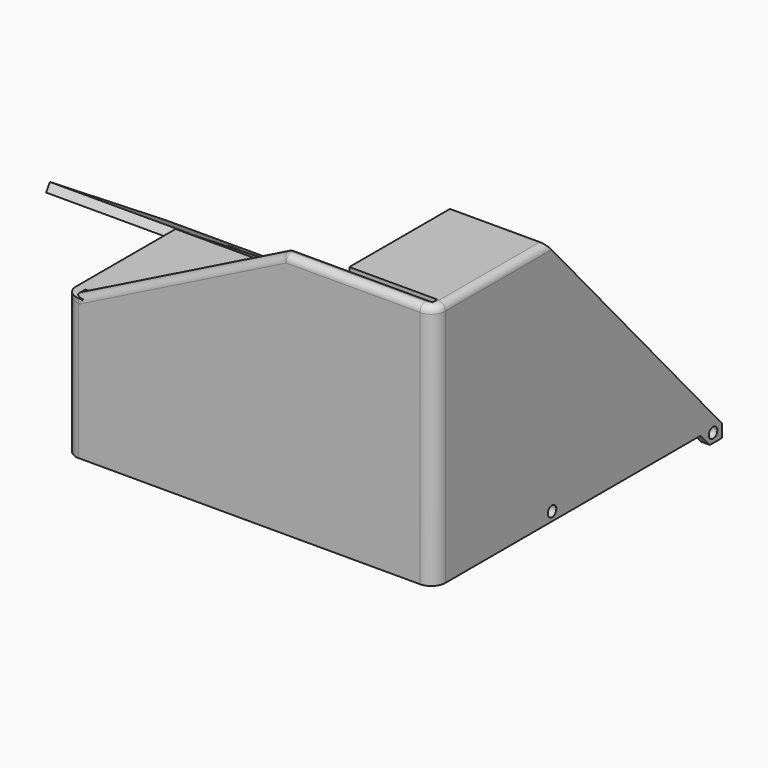
from build123d import *

# Parameters (mm, degrees)
F1_DEPTH      = 3.175
F2_R          = 1.905
F3_DEPTH      = 3.175
F4_R          = 5.08
F5_W          = 45.4158770088
F5_H          = 3.3436195493
F6_DEPTH      = 31.75
F8_DEPTH      = 3.175
F9_W          = 44.698641931
F9_H          = 3.175
F10_DEPTH     = 31.75
F11_R         = 5.08
F13_DEPTH     = 50.8
F14_R         = 1.905
F15_DEPTH     = 25.4
F16_R         = 1.905
F17_DEPTH     = 25.4
F18_T4_DEPTH  = 95.7643351942
F18_T9_DEPTH  = 95.7643351942
F18_S10_R     = 5.08
F18_T11_DEPTH = 50
F19_T1_DEPTH  = 48.2953873372
F19_T3_DEPTH  = 52.07
F19_T5_DEPTH  = 2.1340316571
F19_T10_DEPTH = 2.54
F19_T14_ANGLE = 90


# Not quite as in the source:
# - a fillet or chamfer that OpenCascade refuses, or shapes differently, is made with other operations: its cross-section is extruded or revolved along the edge and cut away or added


with BuildPart() as f1:
    # F0 (on Front) → F1 (new body)
    with BuildSketch(Plane.XZ):
        Polygon((-76.2, 0), (0, 0), (50.8, 0), (50.8, 88.9), (0, 88.9), (-76.2, 50.8), align=None)
    extrude(amount=F1_DEPTH)

    # F2 (on face) → F3 (join)
    with BuildSketch(Plane.YZ.offset(50.8)):
        Polygon((47.625, 88.9), (-3.175, 88.9), (-3.175, 0), (117.0480847359, 0), (121.2547570467, -4.6795206144), (126.6633123159, -4.6795206144), (126.6633123159, 0), align=None)
        with Locations((50.0349625945, 3.2108949963)):
            Circle(F2_R, mode=Mode.SUBTRACT)
        with Locations((122.6691529155, -1.3459949987)):
            Circle(F2_R, mode=Mode.SUBTRACT)
    extrude(amount=F3_DEPTH)

    # F4
    f4_edges = [f1.edges().sort_by_distance(p)[0] for p in [
        (53.975, -3.175, 44.45),
    ]]
    fillet(f4_edges, radius=F4_R)

    # F5 (on face) → F6 (join)
    with BuildSketch(Plane(origin=(50.8, 0, 0), x_dir=(0, -1, 0), z_dir=(-1, 0, 0))):
        with Locations((-24.9170614956, 87.2281902254)):
            Rectangle(F5_W, F5_H)
    extrude(amount=F6_DEPTH)

    # F7 (on face) → F8 (join)
    with BuildSketch(Plane(origin=(-76.2, 0, 0), x_dir=(0, -1, 0), z_dir=(-1, 0, 0))):
        Polygon((-46.908441931, 50.8), (-126.4358460903, 0), (-126.4358460903, -4.5622045459), (-121.1352100604, -4.5622045459), (-113.9930784702, 0), (3.175, 0), (3.175, 50.8), align=None)
    extrude(amount=F8_DEPTH)

    # F9 (on face) → F10 (join)
    with BuildSketch(Plane.YZ.offset(-76.2)):
        with Locations((24.5591209655, 49.2125)):
            Rectangle(F9_W, F9_H)
    extrude(amount=F10_DEPTH)

    # F11
    f11_edges = [f1.edges().sort_by_distance(p)[0] for p in [
        (-79.375, -3.175, 25.4),
    ]]
    fillet(f11_edges, radius=F11_R)

    # F12 (on face) → F13 (join)
    with BuildSketch(Plane(origin=(-79.375, 0, 0), x_dir=(0, -1, 0), z_dir=(-1, 0, 0))):
        Polygon((-51.9476211918, 43.8136345955), (-53.6567879294, 46.4893352632), (-106.1005210159, 12.9896672059), (-104.3913542783, 10.3139665382), align=None)
    extrude(amount=F13_DEPTH)

    # F14 (on face) → F15 (cut)
    with BuildSketch(Plane(origin=(-79.375, 0, 0), x_dir=(0, -1, 0), z_dir=(-1, 0, 0))):
        with Locations((-122.6258460903, -1.2602045459)):
            Circle(F14_R)
        with Locations((-47.4780588517, 3.81)):
            Circle(F14_R)
    extrude(amount=-F15_DEPTH, mode=Mode.SUBTRACT)

    # F16 (on face) → F17 (cut)
    with BuildSketch(Plane(origin=(0, 36.6396759982, 57.359415775), x_dir=(1, 0, 0), z_dir=(0, 0.5383202323, 0.8427403678))):
        with Locations((-83.638317883, 49.4025914339)):
            Circle(F16_R)
    extrude(amount=-F17_DEPTH, mode=Mode.SUBTRACT)

    # F18: fillet of radius 2.54 on 1 edges, made by hand


with BuildPart() as f18_tool2:
    # F18_s3 → F18_t4 (new body)
    with BuildSketch(Plane(origin=(41.2396126628, 0, 20.6198063314), x_dir=(0, 1, 0), z_dir=(-0.894427191, 0, -0.4472135955))):
        with BuildLine():
            ThreePointArc((-3.175, -76.9745772799), (-2.4310512242, -78.7706285041), (-0.635, -79.5145772799))
            Line((-0.635, -79.5145772799), (-3.175, -79.5145772799))
            Line((-3.175, -79.5145772799), (-3.175, -76.9745772799))
        make_face()
    extrude(amount=F18_T4_DEPTH)

    split(bisect_by=Plane.XY.offset(50.8), keep=Keep.TOP)


with BuildPart() as f1_1:
    add(f1.part)

    # F18_t1: cut F18_tool2
    add(f18_tool2.part, mode=Mode.SUBTRACT)


with BuildPart() as f18_tool7:
    # F18_s8 → F18_t9 (new body)
    with BuildSketch(Plane(origin=(41.2396126628, 0, 20.6198063314), x_dir=(0, 1, 0), z_dir=(-0.894427191, 0, -0.4472135955))):
        with BuildLine():
            ThreePointArc((-3.175, -76.9745772799), (-2.4310512242, -78.7706285041), (-0.635, -79.5145772799))
            Line((-0.635, -79.5145772799), (-3.175, -79.5145772799))
            Line((-3.175, -79.5145772799), (-3.175, -76.9745772799))
        make_face()
    extrude(amount=F18_T9_DEPTH)

    # F18_s10 → F18_t11 (cut, symmetric)
    with BuildSketch(Plane.XY.offset(69.2)):
        with Locations((-74.295, 1.905)):
            Circle(F18_S10_R)
    extrude(amount=F18_T11_DEPTH, both=True, mode=Mode.SUBTRACT)


with BuildPart() as f1_2:
    add(f1_1.part)

    # F18_t6: cut F18_tool7
    add(f18_tool7.part, mode=Mode.SUBTRACT)

    # F19: fillet of radius 2.54 on 4 edges, made by hand

    # F19_s2 → F19_t1 (cut)
    with BuildSketch(Plane.YZ.offset(0.5996126628)):
        with BuildLine():
            ThreePointArc((-3.175, 86.36), (-2.4310512242, 88.1560512242), (-0.635, 88.9))
            Line((-0.635, 88.9), (-3.175, 88.9))
            Line((-3.175, 88.9), (-3.175, 86.36))
        make_face()
    extrude(amount=F19_T1_DEPTH, mode=Mode.SUBTRACT)

    # F19_s4 → F19_t3 (cut)
    with BuildSketch(Plane.XZ.offset(-53.975)):
        with BuildLine():
            ThreePointArc((53.975, 86.36), (53.2310512242, 88.1560512242), (51.435, 88.9))
            Line((51.435, 88.9), (53.975, 88.9))
            Line((53.975, 88.9), (53.975, 86.36))
        make_face()
    extrude(amount=F19_T3_DEPTH, mode=Mode.SUBTRACT)

    # F19_s6 → F19_t5 (cut)
    with BuildSketch(Plane.XZ.offset(-1.4990316571)):
        with BuildLine():
            ThreePointArc((0.5996126628, 88.9), (0.0160402447, 88.8320524332), (-0.5363098697, 88.6318450651))
            Line((-0.5363098697, 88.6318450651), (0, 88.9))
            Line((0, 88.9), (0.5996126628, 88.9))
        make_face()
    extrude(amount=F19_T5_DEPTH, mode=Mode.SUBTRACT)


with BuildPart() as f19_tool8:
    # F19_s9 → F19_t10 (new body)
    with BuildSketch(Plane.XZ.offset(0.635)):
        Polygon((0.5996126628, 86.36), (-0.5363098697, 88.6318450651), (0, 88.9), (0.5996126628, 88.9), align=None)
    extrude(amount=F19_T10_DEPTH)

    # F19_s11 → F19_t12 (revolve, cut)
    with BuildSketch(Plane(origin=(0.5996126628, -0.635, 86.36), x_dir=(0.2297529205, 0, -0.9732489895), z_dir=(-0.9732489895, 0, -0.2297529205))):
        with BuildLine():
            ThreePointArc((0, -2.54), (2.54, 0), (0, 2.54))
            Line((0, 2.54), (0, -2.54))
        make_face()
    revolve(axis=Axis((0.5996126628, -0.635, 86.36), (0, -1, 0)), mode=Mode.SUBTRACT)


with BuildPart() as f1_3:
    add(f1_2.part)

    # F19_t7: cut F19_tool8
    add(f19_tool8.part, mode=Mode.SUBTRACT)

    # F19_s13 → F19_t14 (revolve, cut)
    with BuildSketch(Plane.XZ.offset(-1.905)):
        with BuildLine():
            ThreePointArc((53.975, 86.36), (53.2310512242, 88.1560512242), (51.435, 88.9))
            Line((51.435, 88.9), (53.975, 88.9))
            Line((53.975, 88.9), (53.975, 86.36))
        make_face()
    revolve(axis=Axis((48.895, 1.905, 88.9), (0, 0, -1)), revolution_arc=F19_T14_ANGLE, mode=Mode.SUBTRACT)


solid = f1_3.part
